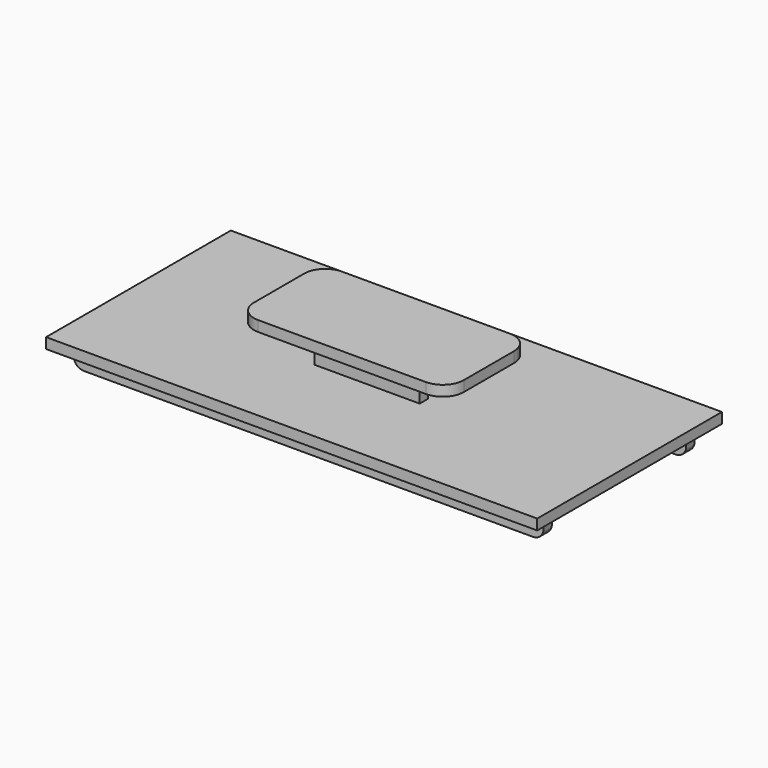
from build123d import *

# Parameters (mm, degrees)
F1_DEPTH  = 5
F7_DEPTH  = 10
F8_R      = 5
F8_2_R    = 5
F9_DEPTH  = 15
F10_DEPTH = 5


# Not quite as in the source:
# - a feature names something its author has since deleted; it is built from what else it names


with BuildPart() as f1:
    # F0 (on Top) → F1 (new body)
    with BuildSketch(Plane.XY):
        Polygon((117, 55), (0, 55), (-117, 55), (-117, -55), (117, -55), align=None)
    extrude(amount=F1_DEPTH)


with BuildPart() as f7:
    # F2 (on Top) → F7 (new body)
    with BuildSketch(Plane.XY):
        Polygon((-112, -40), (-112, -45), (0, -45), (112, -45), (112, -40), align=None)
    extrude(amount=-F7_DEPTH)

    # F8
    f8_edges = [f7.edges().sort_by_distance(p)[0] for p in [
        (-112, -42.5, -10),
        (112, -42.5, -10),
    ]]
    fillet(f8_edges, radius=F8_R)


with BuildPart() as f7b:
    # F2 (on Top) → F7, piece 2 (new body)
    with BuildSketch(Plane.XY):
        Polygon((112, 45), (0, 45), (-112, 45), (-112, 40), (112, 40), align=None)
    extrude(amount=-F7_DEPTH)

    # F8#2
    f8_2_edges = [f7b.edges().sort_by_distance(p)[0] for p in [
        (112, 42.5, -10),
        (-112, 42.5, -10),
    ]]
    fillet(f8_2_edges, radius=F8_2_R)


with BuildPart() as f9:
    # F6 (on offset) → F9 (new body)
    with BuildSketch(Plane.XY.offset(5)):
        Polygon((25, -10), (25, -5), (0, -5), (-25, -5), (-25, -10), align=None)
    extrude(amount=F9_DEPTH)


with BuildPart() as f9b:
    # F6 (on offset) → F9, piece 2 (new body)
    with BuildSketch(Plane.XY.offset(5)):
        Polygon((-25, 5), (0, 5), (25, 5), (25, 10), (-25, 10), align=None)
    extrude(amount=F9_DEPTH)


with BuildPart() as f10:
    # F4 (on offset) → F10 (new body)
    with BuildSketch(Plane.XY.offset(25)):
        with BuildLine():
            Line((40, 25), (0, 25))
            Line((0, 25), (-40, 25))
            ThreePointArc((-40, 25), (-47.0710678119, 22.0710678119), (-50, 15))
            Line((-50, 15), (-50, -15))
            ThreePointArc((-50, -15), (-47.0710678119, -22.0710678119), (-40, -25))
            Line((-40, -25), (40, -25))
            ThreePointArc((40, -25), (47.0710678119, -22.0710678119), (50, -15))
            Line((50, -15), (50, 15))
            ThreePointArc((50, 15), (47.0710678119, 22.0710678119), (40, 25))
        make_face()
    extrude(amount=-F10_DEPTH)


solid = Compound([f1.part, f7.part, f7b.part, f9.part, f9b.part, f10.part])
